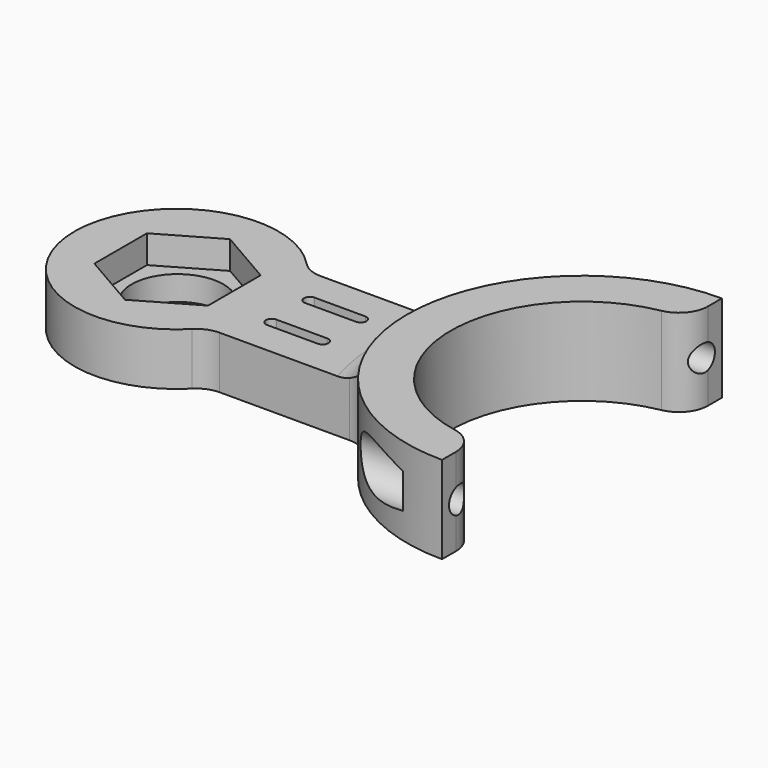
from build123d import *

# Parameters (mm, degrees)
F0_R           = 7.875
F1_DEPTH       = 9
F2_R           = 7.875
F3_DEPTH       = 4.8
F4_DEPTH       = 15
F5_R           = 5
F8_D           = 4.5
F8_DEPTH       = 25
F8_CBORE_D     = 8.25
F8_CBORE_DEPTH = 17
F8_TIP         = 1.3519363928
F11_DEPTH      = 25


# Not quite as in the source:
# - two fillets or chamfers of one size are made in one step


with BuildPart() as f1:
    # F0 (on Top) → F1 (new body)
    with BuildSketch(Plane.XY):
        with BuildLine():
            ThreePointArc((13.8549873727, 10.4671236312), (-17.6653132634, 0.1978340536), (13.609496128, -10.7964352789))
            Line((13.609496128, -10.7964352789), (41.3727938251, -10.7964352789))
            ThreePointArc((41.3727938251, -10.7964352789), (39.3632549532, -0.1760847087), (41.2479854227, 10.4671236312))
            Line((41.2479854227, 10.4671236312), (13.8549873727, 10.4671236312))
        make_face()
        Circle(F0_R, mode=Mode.SUBTRACT)
        with BuildLine():
            ThreePointArc((41.2479854227, 10.4671236312), (39.3632549532, -0.1760847087), (41.3727938251, -10.7964352789))
            ThreePointArc((41.3727938251, -10.7964352789), (52.3906001106, -24.7375530153), (69.362738185, -30))
            Line((69.362738185, -30), (69.362738185, -22.5))
            ThreePointArc((69.362738185, -22.5), (46.862738185, 0), (69.362738185, 22.5))
            Line((69.362738185, 22.5), (69.362738185, 30))
            ThreePointArc((69.362738185, 30), (52.2456956387, 24.6375090963), (41.2479854227, 10.4671236312))
        make_face()
    extrude(amount=F1_DEPTH)

    # F2 (on face) → F3 (cut)
    with BuildSketch(Plane.XY.offset(9)):
        Polygon((9.75, -5.6291651246), (9.75, 5.6291651246), (0, 11.2583302492), (-9.75, 5.6291651246), (-9.75, -5.6291651246), (0, -11.2583302492), align=None)
        Circle(F2_R, mode=Mode.SUBTRACT)
    extrude(amount=-F3_DEPTH, mode=Mode.SUBTRACT)

    # F0 (on Top) → F4 (join)
    with BuildSketch(Plane.XY):
        with BuildLine():
            ThreePointArc((41.2479854227, 10.4671236312), (39.3632549532, -0.1760847087), (41.3727938251, -10.7964352789))
            ThreePointArc((41.3727938251, -10.7964352789), (52.3906001106, -24.7375530153), (69.362738185, -30))
            Line((69.362738185, -30), (69.362738185, -22.5))
            ThreePointArc((69.362738185, -22.5), (46.862738185, 0), (69.362738185, 22.5))
            Line((69.362738185, 22.5), (69.362738185, 30))
            ThreePointArc((69.362738185, 30), (52.2456956387, 24.6375090963), (41.2479854227, 10.4671236312))
        make_face()
    extrude(amount=F4_DEPTH)

    # F5
    f5_edges = [f1.edges().sort_by_distance(p)[0] for p in [
        (13.609496, -10.796435, 4.5),
        (41.247985, 10.467124, 4.5),
        (41.372794, -10.796435, 4.5),
        (39.363255, -0.176085, 9),
        (13.854987, 10.467124, 4.5),
        (69.362738, -22.5, 7.5),
        (69.362738, 22.5, 7.5),
    ]]
    fillet(f5_edges, radius=F5_R)

    # F8
    with Locations(Plane(origin=(44.962738185, 0, 0), x_dir=(0, 1, 0), z_dir=(-1, 0, 0))):
        with Locations((26.25, -7.5), (-26.25, -7.5)):
            CounterBoreHole(F8_D / 2, F8_CBORE_D / 2, F8_CBORE_DEPTH, depth=F8_DEPTH)
            with Locations((0, 0, -(F8_DEPTH + F8_TIP / 2))):  # 118° drill point
                Cone(0, F8_D / 2, F8_TIP, mode=Mode.SUBTRACT)

    # F10 (on face) → F11 (cut)
    with BuildSketch(Plane.XY.offset(9)):
        with BuildLine():
            ThreePointArc((19.4264538586, 5.0838164277), (18.4264538586, 4.0838164277), (19.4264538586, 3.0838164277))
            Line((19.4264538586, 3.0838164277), (28.1441677362, 3.0838164277))
            ThreePointArc((28.1441677362, 3.0838164277), (29.1441677362, 4.0838164277), (28.1441677362, 5.0838164277))
            Line((28.1441677362, 5.0838164277), (19.4264538586, 5.0838164277))
        make_face()
        with BuildLine():
            Line((28.1441677362, -3.0838164277), (19.4264538586, -3.0838164277))
            ThreePointArc((19.4264538586, -3.0838164277), (18.4264538586, -4.0838164277), (19.4264538586, -5.0838164277))
            Line((19.4264538586, -5.0838164277), (28.1441677362, -5.0838164277))
            ThreePointArc((28.1441677362, -5.0838164277), (29.1441677362, -4.0838164277), (28.1441677362, -3.0838164277))
        make_face()
    extrude(amount=-F11_DEPTH, mode=Mode.SUBTRACT)


solid = f1.part
